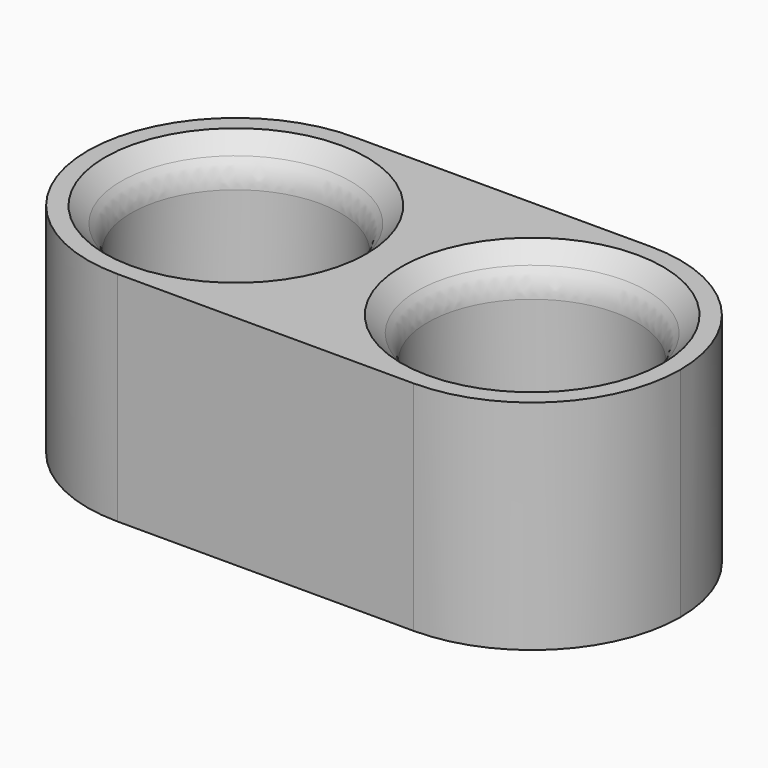
from build123d import *

# Parameters (mm, degrees)
F0_R     = 15.24
F1_DEPTH = 31.75
F2_SIZE  = 3.81
F3_R     = 5.08


# Not quite as in the source:
# - a feature names something its author has since deleted; it is built from what else it names


with BuildPart() as f1:
    # F0 (on Top) → F1 (new body)
    with BuildSketch(Plane.XY):
        with BuildLine():
            ThreePointArc((19.05, -21.59), (34.3164354058, -15.2664354058), (40.64, 0))
            ThreePointArc((40.64, 0), (34.316284436, 15.2665863742), (19.0495729948, 21.5899999958))
            ThreePointArc((19.0495729948, 21.5899999958), (3.7834136258, 15.266284436), (-2.54, 0))
            ThreePointArc((-2.54, 0), (3.7835645942, -15.2664354058), (19.05, -21.59))
        make_face()
        with Locations((19.05, 0)):
            Circle(F0_R, mode=Mode.SUBTRACT)
        with BuildLine():
            Line((-24.13, -21.59), (19.05, -21.59))
            ThreePointArc((19.05, -21.59), (3.7835645942, -15.2664354058), (-2.54, 0))
            ThreePointArc((-2.54, 0), (-8.8635645942, -15.2664354058), (-24.13, -21.59))
        make_face()
        with BuildLine():
            ThreePointArc((-24.13, -21.59), (-8.8635645942, -15.2664354058), (-2.54, 0))
            ThreePointArc((-2.54, 0), (-8.7959724103, 15.1985426235), (-23.9383972097, 21.5891497834))
            ThreePointArc((-23.9383972097, 21.5891497834), (-45.7197874448, 0.0958023383), (-24.13, -21.59))
        make_face()
        with Locations((-24.13, 0)):
            Circle(F0_R, mode=Mode.SUBTRACT)
        with BuildLine():
            ThreePointArc((-2.54, 0), (3.7834136258, 15.266284436), (19.0495729948, 21.5899999958))
            Line((19.0495729948, 21.5899999958), (-23.9383972097, 21.5891497834))
            ThreePointArc((-23.9383972097, 21.5891497834), (-8.7959724103, 15.1985426235), (-2.54, 0))
        make_face()
    extrude(amount=F1_DEPTH)

    # F2
    f2_edges = [f1.edges().sort_by_distance(p)[0] for p in [
        (-39.37, 0, 0),
        (3.81, 0, 0),
        (3.81, 0, 31.75),
        (-39.37, 0, 31.75),
    ]]
    chamfer(f2_edges, length=F2_SIZE)

    # F3
    f3_edges = [f1.edges().sort_by_distance(p)[0] for p in [
        (-39.37, 0, 3.81),
        (-39.37, 0, 27.94),
        (3.81, 0, 27.94),
        (3.81, 0, 3.81),
    ]]
    fillet(f3_edges, radius=F3_R)


solid = f1.part
